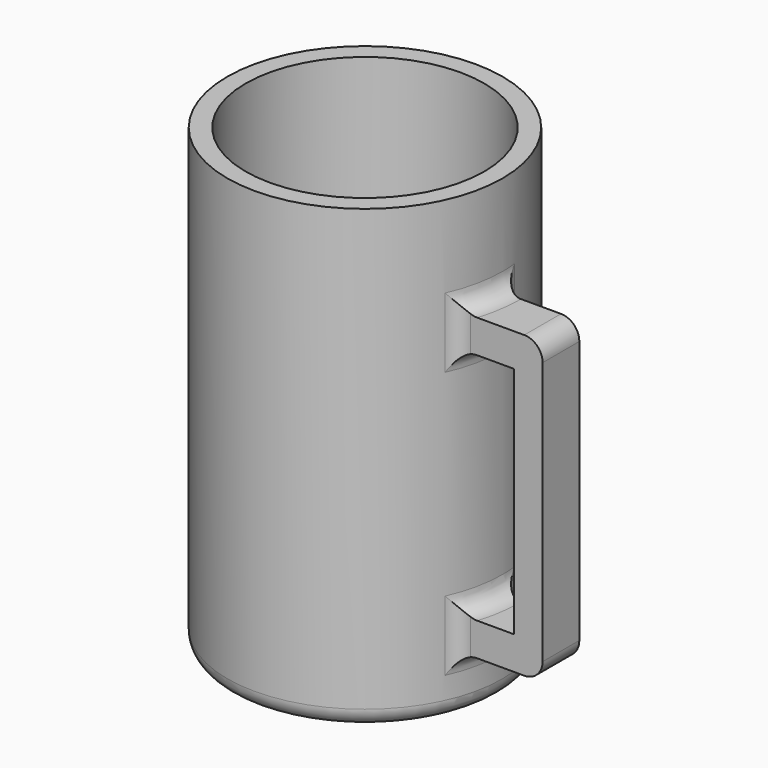
from build123d import *

# Parameters (mm, degrees)
F0_R          = 38.1
F1_DEPTH      = 127
F2_T          = -5.08
F4_DEPTH      = 12.7
F5_T1_DEPTH   = 9.165816009
F5_T3_DEPTH   = 9.165816009
F5_T8_ANGLE   = 38.5701728076
F5_T13_ANGLE  = 38.5701728076
F5_T18_ANGLE  = 38.5701728076
F5_T23_ANGLE  = 38.5701728076
F5_T29_DEPTH  = 17.737031792
F5_T33_ANGLE  = 38.5701728076
F5_T40_ANGLE  = 38.5701728076
F5_T44_DEPTH  = 17.737031792
F5_T51_DEPTH  = 17.737031792
F5_T55_ANGLE  = 38.5701728076
F5_T62_ANGLE  = 38.5701728076
F5_T66_DEPTH  = 17.737031792
F5_T73_ANGLE  = 57.6691249807
F5_T77_DEPTH  = 21.1161541615
F5_T84_ANGLE  = 57.6691249807
F5_T88_DEPTH  = 21.1161541615
F5_T95_ANGLE  = 57.6691249807
F5_T99_DEPTH  = 21.1161541615
F5_T106_ANGLE = 57.6691249807
F5_T110_DEPTH = 21.1161541615
F5_T113_DEPTH = 38.1


# Not quite as in the source:
# - a fillet or chamfer that OpenCascade refuses, or shapes differently, is made with other operations: its cross-section is extruded or revolved along the edge and cut away or added


with BuildPart() as f1:
    # F0 (on Top) → F1 (new body)
    with BuildSketch(Plane.XY):
        Circle(F0_R)
    extrude(amount=F1_DEPTH)

    # F2
    f2_openings = [f1.faces().sort_by_distance(p)[0] for p in [
        (0, 0, 127),
    ]]
    offset(amount=F2_T, openings=f2_openings)

    # F3 (on Front) → F4 (join)
    with BuildSketch(Plane.XZ):
        Polygon((59.3263991177, 99.2357954383), (35.6448739767, 99.2357954383), (35.6448739767, 90.0699794292), (51.4244176447, 90.0699794292), (51.4244176447, 25.3999941051), (35.6448739767, 25.3999941051), (35.6448739767, 16.2341780961), (59.3263991177, 16.2341780961), align=None)
    extrude(amount=F4_DEPTH)

    # F5: fillet of radius 5.08 on 11 edges, made by hand

    # F5_s2 → F5_t1 (join)
    with BuildSketch(Plane.XY.offset(16.2341780961)):
        with BuildLine():
            ThreePointArc((34.720156586, -15.6882352941), (36.5944939832, -13.5119463039), (39.3495107975, -12.7))
            Line((39.3495107975, -12.7), (35.9210244843, -12.7))
            ThreePointArc((35.9210244843, -12.7), (35.3521781973, -14.2068116305), (34.720156586, -15.6882352941))
        make_face()
        with BuildLine():
            ThreePointArc((37.8354134656, 4.4823529412), (39.5059425471, 1.2824713919), (42.880135261, 0))
            Line((42.880135261, 0), (38.1, 0))
            ThreePointArc((38.1, 0), (38.0337958468, 2.2450776113), (37.8354134656, 4.4823529412))
        make_face()
    extrude(amount=F5_T1_DEPTH)

    # F5_s4 → F5_t3 (join)
    with BuildSketch(Plane.XY.offset(90.0699794292)):
        with BuildLine():
            ThreePointArc((34.720156586, -15.6882352941), (36.5944939832, -13.5119463039), (39.3495107975, -12.7))
            Line((39.3495107975, -12.7), (35.9210244843, -12.7))
            ThreePointArc((35.9210244843, -12.7), (35.3521781973, -14.2068116305), (34.720156586, -15.6882352941))
        make_face()
        with BuildLine():
            ThreePointArc((37.8354134656, 4.4823529412), (39.5059425471, 1.2824713919), (42.880135261, 0))
            Line((42.880135261, 0), (38.1, 0))
            ThreePointArc((38.1, 0), (38.0337958468, 2.2450776113), (37.8354134656, 4.4823529412))
        make_face()
    extrude(amount=F5_T3_DEPTH)


with BuildPart() as f5_tool6:
    # F5_s7 → F5_t8 (revolve)
    with BuildSketch(Plane.XZ):
        with BuildLine():
            ThreePointArc((38.1, 104.3157954383), (39.5878975516, 100.7236929899), (43.18, 99.2357954383))
            Line((43.18, 99.2357954383), (38.1, 99.2357954383))
            Line((38.1, 99.2357954383), (38.1, 104.3157954383))
        make_face()
    revolve(axis=Axis((0, 0, 99.2357954383), (0, 0, -1)), revolution_arc=F5_T8_ANGLE)

    split(bisect_by=Plane.XZ.offset(12.7), keep=Keep.BOTTOM)


with BuildPart() as f1_1:
    add(f1.part)

    # F5_t5: union F5_tool6
    add(f5_tool6.part)


with BuildPart() as f5_tool11:
    # F5_s12 → F5_t13 (revolve)
    with BuildSketch(Plane.XZ):
        with BuildLine():
            ThreePointArc((38.1, 84.9899794292), (39.5878975516, 88.5820818777), (43.18, 90.0699794292))
            Line((43.18, 90.0699794292), (38.1, 90.0699794292))
            Line((38.1, 90.0699794292), (38.1, 84.9899794292))
        make_face()
    revolve(axis=Axis((0, 0, 90.0699794292), (0, 0, -1)), revolution_arc=F5_T13_ANGLE)

    split(bisect_by=Plane.XZ.offset(12.7), keep=Keep.BOTTOM)


with BuildPart() as f1_2:
    add(f1_1.part)

    # F5_t10: union F5_tool11
    add(f5_tool11.part)


with BuildPart() as f5_tool16:
    # F5_s17 → F5_t18 (revolve)
    with BuildSketch(Plane.XZ):
        with BuildLine():
            ThreePointArc((38.1, 11.1541780961), (39.5878975516, 14.7462805445), (43.18, 16.2341780961))
            Line((43.18, 16.2341780961), (38.1, 16.2341780961))
            Line((38.1, 16.2341780961), (38.1, 11.1541780961))
        make_face()
    revolve(axis=Axis((0, 0, 16.2341780961), (0, 0, -1)), revolution_arc=F5_T18_ANGLE)

    split(bisect_by=Plane.XZ.offset(12.7), keep=Keep.BOTTOM)


with BuildPart() as f1_3:
    add(f1_2.part)

    # F5_t15: union F5_tool16
    add(f5_tool16.part)


with BuildPart() as f5_tool21:
    # F5_s22 → F5_t23 (revolve)
    with BuildSketch(Plane.XZ):
        with BuildLine():
            ThreePointArc((38.1, 30.4799941051), (39.5878975516, 26.8878916567), (43.18, 25.3999941051))
            Line((43.18, 25.3999941051), (38.1, 25.3999941051))
            Line((38.1, 25.3999941051), (38.1, 30.4799941051))
        make_face()
    revolve(axis=Axis((0, 0, 25.3999941051), (0, 0, -1)), revolution_arc=F5_T23_ANGLE)

    split(bisect_by=Plane.XZ.offset(12.7), keep=Keep.BOTTOM)


with BuildPart() as f1_4:
    add(f1_3.part)

    # F5_t20: union F5_tool21
    add(f5_tool21.part)


with BuildPart() as f5_tool27:
    # F5_s28 → F5_t29 (new body)
    with BuildSketch(Plane.XY.offset(33.9712098881)):
        with BuildLine():
            ThreePointArc((34.720156586, -15.6882352941), (36.5944939832, -13.5119463039), (39.3495107975, -12.7))
            Line((39.3495107975, -12.7), (35.9210244843, -12.7))
            ThreePointArc((35.9210244843, -12.7), (35.3521781973, -14.2068116305), (34.720156586, -15.6882352941))
        make_face()
    extrude(amount=-F5_T29_DEPTH)

    split(bisect_by=Plane.XY.offset(25.3999941051), keep=Keep.TOP)


with BuildPart() as f5_tool31:
    # F5_s32 → F5_t33 (revolve)
    with BuildSketch(Plane.XZ):
        with BuildLine():
            ThreePointArc((38.1, 30.4799941051), (39.5878975516, 26.8878916567), (43.18, 25.3999941051))
            Line((43.18, 25.3999941051), (38.1, 25.3999941051))
            Line((38.1, 25.3999941051), (38.1, 30.4799941051))
        make_face()
    revolve(axis=Axis((0, 0, 25.3999941051), (0, 0, -1)), revolution_arc=F5_T33_ANGLE)

    split(bisect_by=Plane.XZ.offset(12.7), keep=Keep.TOP)


with BuildPart() as f5_tool27_1:
    add(f5_tool27.part)

    # F5_t35: intersect F5_tool31
    add(f5_tool31.part, mode=Mode.INTERSECT)


with BuildPart() as f1_5:
    add(f1_4.part)

    # F5_t25: union F5_tool27
    add(f5_tool27_1.part)


with BuildPart() as f5_tool38:
    # F5_s39 → F5_t40 (revolve)
    with BuildSketch(Plane.XZ):
        with BuildLine():
            ThreePointArc((38.1, 11.1541780961), (39.5878975516, 14.7462805445), (43.18, 16.2341780961))
            Line((43.18, 16.2341780961), (38.1, 16.2341780961))
            Line((38.1, 16.2341780961), (38.1, 11.1541780961))
        make_face()
    revolve(axis=Axis((0, 0, 16.2341780961), (0, 0, -1)), revolution_arc=F5_T40_ANGLE)

    split(bisect_by=Plane.XZ.offset(12.7), keep=Keep.TOP)


with BuildPart() as f5_tool42:
    # F5_s43 → F5_t44 (new body)
    with BuildSketch(Plane.XY.offset(25.3999941051)):
        with BuildLine():
            ThreePointArc((34.720156586, -15.6882352941), (36.5944939832, -13.5119463039), (39.3495107975, -12.7))
            Line((39.3495107975, -12.7), (35.9210244843, -12.7))
            ThreePointArc((35.9210244843, -12.7), (35.3521781973, -14.2068116305), (34.720156586, -15.6882352941))
        make_face()
    extrude(amount=-F5_T44_DEPTH)

    split(bisect_by=Plane.XY.offset(16.2341780961), keep=Keep.BOTTOM)


with BuildPart() as f5_tool38_1:
    add(f5_tool38.part)

    # F5_t46: intersect F5_tool42
    add(f5_tool42.part, mode=Mode.INTERSECT)


with BuildPart() as f1_6:
    add(f1_5.part)

    # F5_t36: union F5_tool38
    add(f5_tool38_1.part)


with BuildPart() as f5_tool49:
    # F5_s50 → F5_t51 (new body)
    with BuildSketch(Plane.XY.offset(107.8070112213)):
        with BuildLine():
            ThreePointArc((34.720156586, -15.6882352941), (36.5944939832, -13.5119463039), (39.3495107975, -12.7))
            Line((39.3495107975, -12.7), (35.9210244843, -12.7))
            ThreePointArc((35.9210244843, -12.7), (35.3521781973, -14.2068116305), (34.720156586, -15.6882352941))
        make_face()
    extrude(amount=-F5_T51_DEPTH)

    split(bisect_by=Plane.XY.offset(99.2357954383), keep=Keep.TOP)


with BuildPart() as f5_tool53:
    # F5_s54 → F5_t55 (revolve)
    with BuildSketch(Plane.XZ):
        with BuildLine():
            ThreePointArc((38.1, 104.3157954383), (39.5878975516, 100.7236929899), (43.18, 99.2357954383))
            Line((43.18, 99.2357954383), (38.1, 99.2357954383))
            Line((38.1, 99.2357954383), (38.1, 104.3157954383))
        make_face()
    revolve(axis=Axis((0, 0, 99.2357954383), (0, 0, -1)), revolution_arc=F5_T55_ANGLE)

    split(bisect_by=Plane.XZ.offset(12.7), keep=Keep.TOP)


with BuildPart() as f5_tool49_1:
    add(f5_tool49.part)

    # F5_t57: intersect F5_tool53
    add(f5_tool53.part, mode=Mode.INTERSECT)


with BuildPart() as f1_7:
    add(f1_6.part)

    # F5_t47: union F5_tool49
    add(f5_tool49_1.part)


with BuildPart() as f5_tool60:
    # F5_s61 → F5_t62 (revolve)
    with BuildSketch(Plane.XZ):
        with BuildLine():
            ThreePointArc((38.1, 84.9899794292), (39.5878975516, 88.5820818777), (43.18, 90.0699794292))
            Line((43.18, 90.0699794292), (38.1, 90.0699794292))
            Line((38.1, 90.0699794292), (38.1, 84.9899794292))
        make_face()
    revolve(axis=Axis((0, 0, 90.0699794292), (0, 0, -1)), revolution_arc=F5_T62_ANGLE)

    split(bisect_by=Plane.XZ.offset(12.7), keep=Keep.TOP)


with BuildPart() as f5_tool64:
    # F5_s65 → F5_t66 (new body)
    with BuildSketch(Plane.XY.offset(99.2357954383)):
        with BuildLine():
            ThreePointArc((34.720156586, -15.6882352941), (36.5944939832, -13.5119463039), (39.3495107975, -12.7))
            Line((39.3495107975, -12.7), (35.9210244843, -12.7))
            ThreePointArc((35.9210244843, -12.7), (35.3521781973, -14.2068116305), (34.720156586, -15.6882352941))
        make_face()
    extrude(amount=-F5_T66_DEPTH)

    split(bisect_by=Plane.XY.offset(90.0699794292), keep=Keep.BOTTOM)


with BuildPart() as f5_tool60_1:
    add(f5_tool60.part)

    # F5_t68: intersect F5_tool64
    add(f5_tool64.part, mode=Mode.INTERSECT)


with BuildPart() as f1_8:
    add(f1_7.part)

    # F5_t58: union F5_tool60
    add(f5_tool60_1.part)


with BuildPart() as f5_tool71:
    # F5_s72 → F5_t73 (revolve)
    with BuildSketch(Plane(origin=(0, 0, 0), x_dir=(0, 0, 1), z_dir=(-0.3272006177, 0.9449548962, 0))):
        with BuildLine():
            ThreePointArc((104.3157954383, 38.1), (100.7236929899, 39.5878975516), (99.2357954383, 43.18))
            Line((99.2357954383, 43.18), (99.2357954383, 38.1))
            Line((99.2357954383, 38.1), (104.3157954383, 38.1))
        make_face()
    revolve(axis=Axis((0, 0, 99.2357954383), (0, 0, -1)), revolution_arc=F5_T73_ANGLE)

    split(bisect_by=Plane.XZ, keep=Keep.BOTTOM)


with BuildPart() as f5_tool75:
    # F5_s76 → F5_t77 (new body)
    with BuildSketch(Plane.XY.offset(90.0699794292)):
        with BuildLine():
            ThreePointArc((37.8354134656, 4.4823529412), (39.5059425471, 1.2824713919), (42.880135261, 0))
            Line((42.880135261, 0), (38.1, 0))
            ThreePointArc((38.1, 0), (38.0337958468, 2.2450776113), (37.8354134656, 4.4823529412))
        make_face()
    extrude(amount=F5_T77_DEPTH)

    split(bisect_by=Plane.XY.offset(99.2357954383), keep=Keep.TOP)


with BuildPart() as f5_tool71_1:
    add(f5_tool71.part)

    # F5_t79: intersect F5_tool75
    add(f5_tool75.part, mode=Mode.INTERSECT)


with BuildPart() as f1_9:
    add(f1_8.part)

    # F5_t69: union F5_tool71
    add(f5_tool71_1.part)


with BuildPart() as f5_tool82:
    # F5_s83 → F5_t84 (revolve)
    with BuildSketch(Plane(origin=(0, 0, 0), x_dir=(0, 0, 1), z_dir=(-0.3272006177, 0.9449548962, 0))):
        with BuildLine():
            ThreePointArc((84.9899794292, 38.1), (88.5820818777, 39.5878975516), (90.0699794292, 43.18))
            Line((90.0699794292, 43.18), (90.0699794292, 38.1))
            Line((90.0699794292, 38.1), (84.9899794292, 38.1))
        make_face()
    revolve(axis=Axis((0, 0, 90.0699794292), (0, 0, -1)), revolution_arc=F5_T84_ANGLE)

    split(bisect_by=Plane.XZ, keep=Keep.BOTTOM)


with BuildPart() as f5_tool86:
    # F5_s87 → F5_t88 (new body)
    with BuildSketch(Plane.XY.offset(78.1196412768)):
        with BuildLine():
            ThreePointArc((37.8354134656, 4.4823529412), (39.5059425471, 1.2824713919), (42.880135261, 0))
            Line((42.880135261, 0), (38.1, 0))
            ThreePointArc((38.1, 0), (38.0337958468, 2.2450776113), (37.8354134656, 4.4823529412))
        make_face()
    extrude(amount=F5_T88_DEPTH)

    split(bisect_by=Plane.XY.offset(90.0699794292), keep=Keep.BOTTOM)


with BuildPart() as f5_tool82_1:
    add(f5_tool82.part)

    # F5_t90: intersect F5_tool86
    add(f5_tool86.part, mode=Mode.INTERSECT)


with BuildPart() as f1_10:
    add(f1_9.part)

    # F5_t80: union F5_tool82
    add(f5_tool82_1.part)


with BuildPart() as f5_tool93:
    # F5_s94 → F5_t95 (revolve)
    with BuildSketch(Plane(origin=(0, 0, 0), x_dir=(0, 0, 1), z_dir=(-0.3272006177, 0.9449548962, 0))):
        with BuildLine():
            ThreePointArc((11.1541780961, 38.1), (14.7462805445, 39.5878975516), (16.2341780961, 43.18))
            Line((16.2341780961, 43.18), (16.2341780961, 38.1))
            Line((16.2341780961, 38.1), (11.1541780961, 38.1))
        make_face()
    revolve(axis=Axis((0, 0, 16.2341780961), (0, 0, -1)), revolution_arc=F5_T95_ANGLE)

    split(bisect_by=Plane.XZ, keep=Keep.BOTTOM)


with BuildPart() as f5_tool97:
    # F5_s98 → F5_t99 (new body)
    with BuildSketch(Plane.XY.offset(4.2838399436)):
        with BuildLine():
            ThreePointArc((37.8354134656, 4.4823529412), (39.5059425471, 1.2824713919), (42.880135261, 0))
            Line((42.880135261, 0), (38.1, 0))
            ThreePointArc((38.1, 0), (38.0337958468, 2.2450776113), (37.8354134656, 4.4823529412))
        make_face()
    extrude(amount=F5_T99_DEPTH)

    split(bisect_by=Plane.XY.offset(16.2341780961), keep=Keep.BOTTOM)


with BuildPart() as f5_tool93_1:
    add(f5_tool93.part)

    # F5_t101: intersect F5_tool97
    add(f5_tool97.part, mode=Mode.INTERSECT)


with BuildPart() as f1_11:
    add(f1_10.part)

    # F5_t91: union F5_tool93
    add(f5_tool93_1.part)


with BuildPart() as f5_tool104:
    # F5_s105 → F5_t106 (revolve)
    with BuildSketch(Plane(origin=(0, 0, 0), x_dir=(0, 0, 1), z_dir=(-0.3272006177, 0.9449548962, 0))):
        with BuildLine():
            ThreePointArc((30.4799941051, 38.1), (26.8878916567, 39.5878975516), (25.3999941051, 43.18))
            Line((25.3999941051, 43.18), (25.3999941051, 38.1))
            Line((25.3999941051, 38.1), (30.4799941051, 38.1))
        make_face()
    revolve(axis=Axis((0, 0, 25.3999941051), (0, 0, -1)), revolution_arc=F5_T106_ANGLE)

    split(bisect_by=Plane.XZ, keep=Keep.BOTTOM)


with BuildPart() as f5_tool108:
    # F5_s109 → F5_t110 (new body)
    with BuildSketch(Plane.XY.offset(16.2341780961)):
        with BuildLine():
            ThreePointArc((37.8354134656, 4.4823529412), (39.5059425471, 1.2824713919), (42.880135261, 0))
            Line((42.880135261, 0), (38.1, 0))
            ThreePointArc((38.1, 0), (38.0337958468, 2.2450776113), (37.8354134656, 4.4823529412))
        make_face()
    extrude(amount=F5_T110_DEPTH)

    split(bisect_by=Plane.XY.offset(25.3999941051), keep=Keep.TOP)


with BuildPart() as f5_tool104_1:
    add(f5_tool104.part)

    # F5_t112: intersect F5_tool108
    add(f5_tool108.part, mode=Mode.INTERSECT)


with BuildPart() as f1_12:
    add(f1_11.part)

    # F5_t102: union F5_tool104
    add(f5_tool104_1.part)

    # F5_s114 → F5_t113 (cut)
    with BuildSketch(Plane.XZ.offset(-12.7)):
        with BuildLine():
            ThreePointArc((59.3263991177, 94.1557954383), (57.8385015661, 97.7478978867), (54.2463991177, 99.2357954383))
            Line((54.2463991177, 99.2357954383), (59.3263991177, 99.2357954383))
            Line((59.3263991177, 99.2357954383), (59.3263991177, 94.1557954383))
        make_face()
        with BuildLine():
            ThreePointArc((54.2463991177, 16.2341780961), (57.8385015661, 17.7220756476), (59.3263991177, 21.3141780961))
            Line((59.3263991177, 21.3141780961), (59.3263991177, 16.2341780961))
            Line((59.3263991177, 16.2341780961), (54.2463991177, 16.2341780961))
        make_face()
    extrude(amount=F5_T113_DEPTH, mode=Mode.SUBTRACT)

    # F5_s115 → F5_t116 (revolve, cut)
    with BuildSketch(Plane.XZ):
        with BuildLine():
            ThreePointArc((38.1, 5.08), (36.6121024484, 1.4878975516), (33.02, 0))
            Line((33.02, 0), (38.1, 0))
            Line((38.1, 0), (38.1, 5.08))
        make_face()
    revolve(axis=Axis((0, 0, 0), (0, 0, 1)), mode=Mode.SUBTRACT)


solid = f1_12.part
